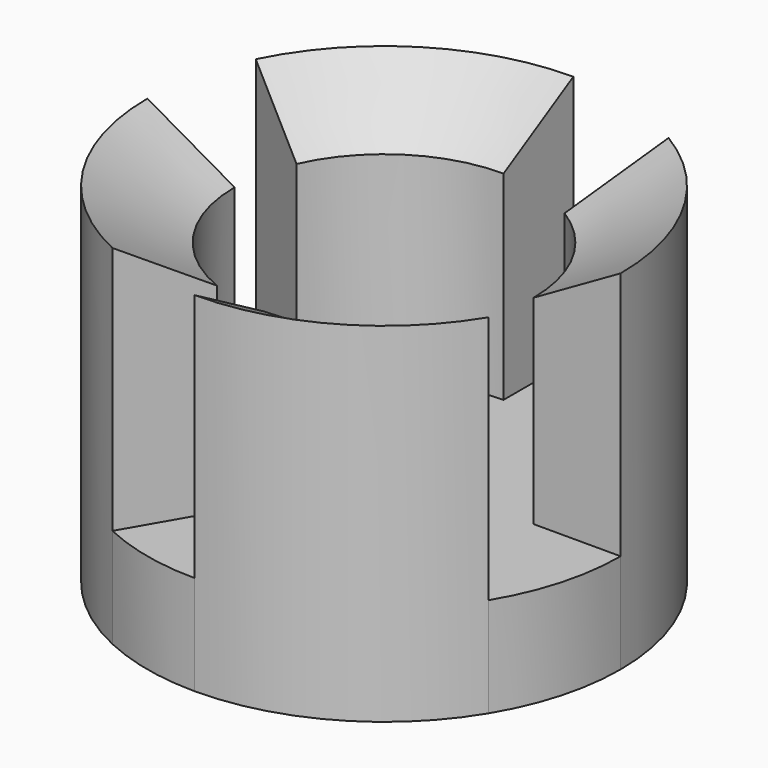
from build123d import *

# Parameters (mm, degrees)
F1_DEPTH   = 2
F2_DEPTH   = 7
F3_SIZE2   = 1.74999
F3_SIZE    = 0.99999
F3_2_SIZE2 = 1.74999
F3_2_SIZE  = 0.99999
F3_3_SIZE2 = 1.74999
F3_3_SIZE  = 0.99999
F3_4_SIZE2 = 1.74999
F3_4_SIZE  = 0.99999


# Not quite as in the source:
# - a fillet or chamfer is up to 0.001 mm smaller than in the source, because OpenCascade refuses the exact size


with BuildPart() as f1:
    # F0 (on Top) → F1 (new body)
    with BuildSketch(Plane.XY):
        with BuildLine():
            ThreePointArc((2.5497759502, -1.5807095255), (2.8852493697, -0.8217883394), (3, 0))
            ThreePointArc((3, 0), (2.6235481729, 1.4549896853), (1.5886700104, 2.544823687))
            ThreePointArc((1.5886700104, 2.544823687), (0.8262956308, 2.8839617769), (0, 3))
            ThreePointArc((0, 3), (-1.6310845521, 2.51784892), (-2.7378829853, 1.226375456))
            ThreePointArc((-2.7378829853, 1.226375456), (-2.9337389928, 0.6270370979), (-3, 0))
            ThreePointArc((-3, 0), (-2.488818496, -1.6750470125), (-1.1294783373, -2.7792586575))
            ThreePointArc((-1.1294783373, -2.7792586575), (-0.5754233343, -2.944297537), (0, -3))
            ThreePointArc((0, -3), (1.4590872872, -2.6212715022), (2.5497759502, -1.5807095255))
        make_face()
        with BuildLine():
            Line((0, -4.75), (0, -3))
            ThreePointArc((0, -3), (-0.5754233343, -2.944297537), (-1.1294783373, -2.7792586575))
            Line((-1.1294783373, -2.7792586575), (-2.0097266443, -4.3038934484))
            ThreePointArc((-2.0097266443, -4.3038934484), (-1.0293216504, -4.6371324048), (0, -4.75))
        make_face()
        with BuildLine():
            Line((4.75, 0), (3, 0))
            ThreePointArc((3, 0), (2.8852493697, -0.8217883394), (2.5497759502, -1.5807095255))
            Line((2.5497759502, -1.5807095255), (4.0657909798, -2.455981211))
            ThreePointArc((4.0657909798, -2.455981211), (4.5757516953, -1.2747534754), (4.75, 0))
        make_face()
        with BuildLine():
            ThreePointArc((-3, 0), (-2.9337389928, 0.6270370979), (-2.7378829853, 1.226375456))
            Line((-2.7378829853, 1.226375456), (-4.2584618162, 2.1042820533))
            ThreePointArc((-4.2584618162, 2.1042820533), (-4.625483414, 1.0804643384), (-4.75, 0))
            Line((-4.75, 0), (-3, 0))
        make_face()
        with BuildLine():
            ThreePointArc((0, 3), (0.8262956308, 2.8839617769), (1.5886700104, 2.544823687))
            Line((1.5886700104, 2.544823687), (2.4639985646, 4.0609372162))
            ThreePointArc((2.4639985646, 4.0609372162), (1.2792670212, 4.5744918722), (0, 4.75))
            Line((0, 4.75), (0, 3))
        make_face()
    extrude(amount=F1_DEPTH)

    # F0 (on Top) → F2 (join)
    with BuildSketch(Plane.XY):
        with BuildLine():
            Line((-2.0097266443, -4.3038934484), (-1.1294783373, -2.7792586575))
            ThreePointArc((-1.1294783373, -2.7792586575), (-2.488818496, -1.6750470125), (-3, 0))
            Line((-3, 0), (-4.75, 0))
            ThreePointArc((-4.75, 0), (-4.0067880877, -2.5511074497), (-2.0097266443, -4.3038934484))
        make_face()
        with BuildLine():
            Line((4.0657909798, -2.455981211), (2.5497759502, -1.5807095255))
            ThreePointArc((2.5497759502, -1.5807095255), (1.4590872872, -2.6212715022), (0, -3))
            Line((0, -3), (0, -4.75))
            ThreePointArc((0, -4.75), (2.334158226, -4.1369318795), (4.0657909798, -2.455981211))
        make_face()
        with BuildLine():
            ThreePointArc((1.5886700104, 2.544823687), (2.6235481729, 1.4549896853), (3, 0))
            Line((3, 0), (4.75, 0))
            ThreePointArc((4.75, 0), (4.1392326089, 2.3300758376), (2.4639985646, 4.0609372162))
            Line((2.4639985646, 4.0609372162), (1.5886700104, 2.544823687))
        make_face()
        with BuildLine():
            ThreePointArc((-2.7378829853, 1.226375456), (-1.6310845521, 2.51784892), (0, 3))
            Line((0, 3), (0, 4.75))
            ThreePointArc((0, 4.75), (-2.5067070278, 4.0347143488), (-4.2584618162, 2.1042820533))
            Line((-4.2584618162, 2.1042820533), (-2.7378829853, 1.226375456))
        make_face()
    extrude(amount=F2_DEPTH)

    # F3 (size 1 and 1.75 in the source; OpenCascade refuses exactly that, so slightly less here)
    f3_edges = [f1.edges().sort_by_distance(p)[0] for p in [
        (-2.488818, -1.675047, 7),
    ]]
    f3_side = f1.faces().sort_by_distance((-2.488818, -1.675047, 4.5))[0]
    chamfer(f3_edges, length=F3_SIZE, length2=F3_SIZE2, reference=f3_side)

    # F3#2 (size 1 and 1.75 in the source; OpenCascade refuses exactly that, so slightly less here)
    f3_2_edges = [f1.edges().sort_by_distance(p)[0] for p in [
        (-1.631085, 2.517849, 7),
    ]]
    f3_2_side = f1.faces().sort_by_distance((-1.631085, 2.517849, 4.5))[0]
    chamfer(f3_2_edges, length=F3_2_SIZE, length2=F3_2_SIZE2, reference=f3_2_side)

    # F3#3 (size 1 and 1.75 in the source; OpenCascade refuses exactly that, so slightly less here)
    f3_3_edges = [f1.edges().sort_by_distance(p)[0] for p in [
        (2.623548, 1.45499, 7),
    ]]
    f3_3_side = f1.faces().sort_by_distance((2.623548, 1.45499, 4.5))[0]
    chamfer(f3_3_edges, length=F3_3_SIZE, length2=F3_3_SIZE2, reference=f3_3_side)

    # F3#4 (size 1 and 1.75 in the source; OpenCascade refuses exactly that, so slightly less here)
    f3_4_edges = [f1.edges().sort_by_distance(p)[0] for p in [
        (1.459087, -2.621272, 7),
    ]]
    f3_4_side = f1.faces().sort_by_distance((1.459087, -2.621272, 4.5))[0]
    chamfer(f3_4_edges, length=F3_4_SIZE, length2=F3_4_SIZE2, reference=f3_4_side)


solid = f1.part
